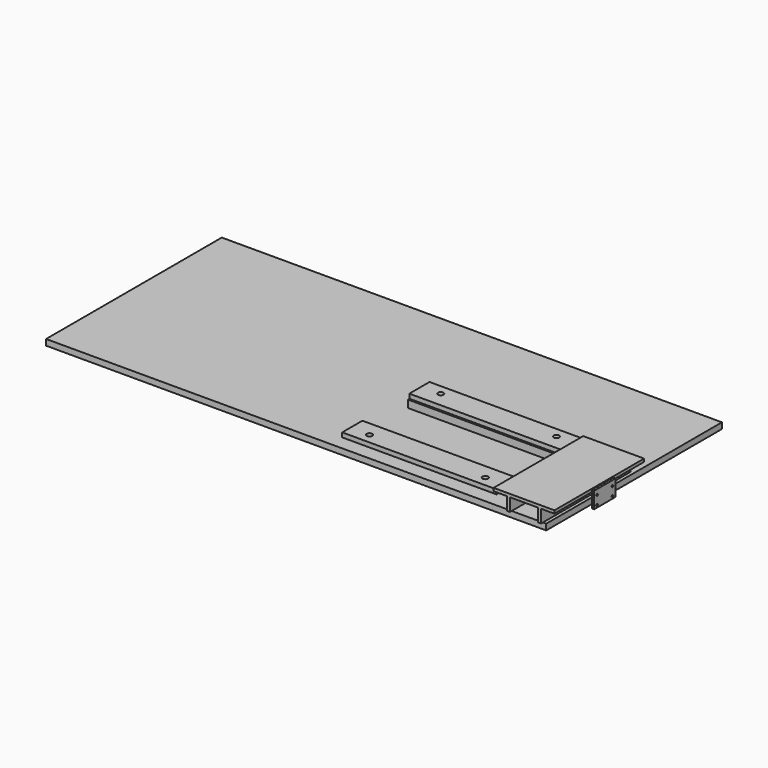
from build123d import *

# Parameters (mm, degrees)
F0_W      = 4279.9
F0_H      = 1879.6
F1_DEPTH  = 50.8
F2_W      = 1320.8
F2_H      = 31.75
F3_DEPTH  = 63.5
F4_W      = 1320.8
F4_H      = 215.9
F5_DEPTH  = 38.1
F7_D      = 47.625
F7_DEPTH  = 50.8
F7_TIP    = 14.3079934906
F8_W      = 25.4
F8_H      = 958.85
F9_DEPTH  = 111.252
F10_W     = 520.7
F10_H     = 958.85
F11_DEPTH = 25.4
F12_W     = 228.6
F12_H     = 139.7
F13_DEPTH = 19.05
F15_D     = 17.4625
F15_DEPTH = 50.8
F15_TIP   = 5.2462642799


# Not quite as in the source:
# - a length typed as a fraction of an inch, garbled in the dataset ("3 / 203.2 mm" for 3/8 in), is restored


with BuildPart() as f1:
    # F0 (on Top) → F1 (new body)
    with BuildSketch(Plane.XY):
        Rectangle(F0_W, F0_H)
    extrude(amount=-F1_DEPTH)

    # F2 (on face) → F3 (join)
    with BuildSketch(Plane.XY):
        with Locations((1031.875, -695.325)):
            Rectangle(F2_W, F2_H)
        with Locations((1031.875, -193.675)):
            Rectangle(F2_W, F2_H)
    extrude(amount=F3_DEPTH)

    # F4 (on face) → F5 (join)
    with BuildSketch(Plane.XY.offset(63.5)):
        with Locations((1031.875, -803.402)):
            Rectangle(F4_W, F4_H)
        with Locations((1031.875, -85.598)):
            Rectangle(F4_W, F4_H)
    extrude(amount=F5_DEPTH)

    # F7
    with Locations(Plane.XY.offset(101.6)):
        with Locations((536.575, -63.5), (1527.175, -63.5), (536.575, -825.5), (1527.175, -825.5)):
            Hole(F7_D / 2, depth=F7_DEPTH)
            with Locations((0, 0, -(F7_DEPTH + F7_TIP / 2))):  # 118° drill point
                Cone(0, F7_D / 2, F7_TIP, mode=Mode.SUBTRACT)

    # F8 (on face) → F9 (join)
    with BuildSketch(Plane.XY):
        with Locations((1831.975, -479.425)):
            Rectangle(F8_W, F8_H)
        with Locations((2098.675, -479.425)):
            Rectangle(F8_W, F8_H)
    extrude(amount=F9_DEPTH)

    # F10 (on face) → F11 (join)
    with BuildSketch(Plane.XY.offset(111.252)):
        with Locations((1965.325, -479.425)):
            Rectangle(F10_W, F10_H)
    extrude(amount=F11_DEPTH)

    # F12 (on face) → F13 (join)
    with BuildSketch(Plane.YZ.offset(2225.675)):
        with Locations((-444.5, 57.15)):
            Rectangle(F12_W, F12_H)
    extrude(amount=F13_DEPTH)

    # F15
    with Locations(Plane.YZ.offset(2244.725)):
        with Locations((-527.05, 82.804), (-527.05, 6.604), (-361.95, 6.604), (-361.95, 82.804)):
            Hole(F15_D / 2, depth=F15_DEPTH)
            with Locations((0, 0, -(F15_DEPTH + F15_TIP / 2))):  # 118° drill point
                Cone(0, F15_D / 2, F15_TIP, mode=Mode.SUBTRACT)


solid = f1.part
